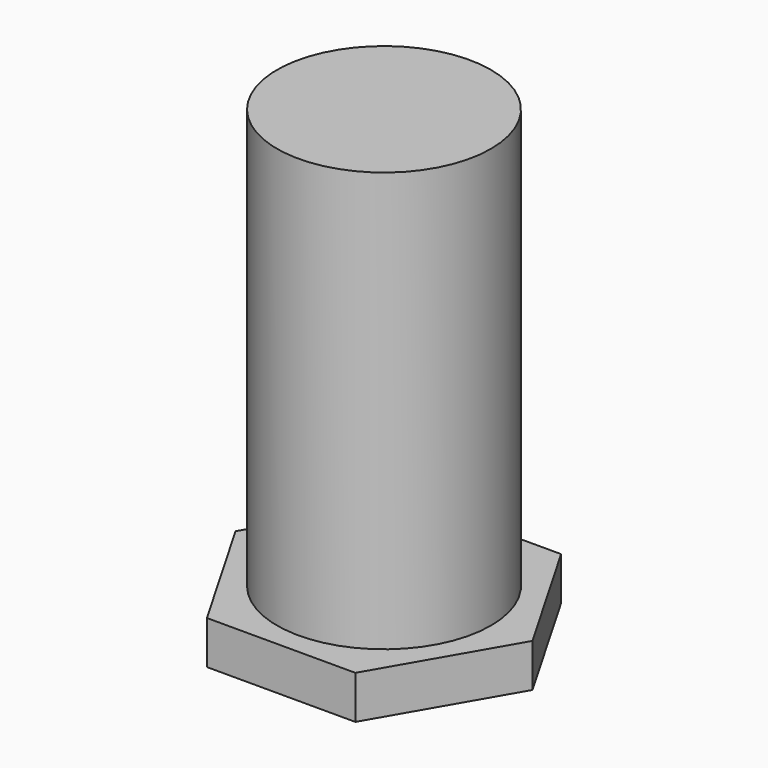
from build123d import *

# Parameters (mm, degrees)
F1_DEPTH = 1.6002
F2_R     = 3.9624
F3_DEPTH = 15.5448
F5_D     = 4.7244
F5_DEPTH = 10.922
F5_TIP   = 1.4193529543


# Not quite as in the source:
# - a feature names something its author has since deleted; it is built from what else it names


with BuildPart() as f1:
    # F0 (on Top) → F1 (new body)
    with BuildSketch(Plane.XY):
        Polygon((5.4991, 0), (2.74955, 4.762360298), (-2.74955, 4.762360298), (-5.4991, 0), (-2.74955, -4.762360298), (2.74955, -4.762360298), align=None)
    extrude(amount=F1_DEPTH)

    # F2 (on face) → F3 (join)
    with BuildSketch(Plane.XY.offset(1.6002)):
        Circle(F2_R)
    extrude(amount=F3_DEPTH)

    # F5
    with Locations(Plane(origin=(0, 0, 0), x_dir=(1, 0, 0), z_dir=(0, 0, -1))):
        with Locations((0, 0)):
            Hole(F5_D / 2, depth=F5_DEPTH)
            with Locations((0, 0, -(F5_DEPTH + F5_TIP / 2))):  # 118° drill point
                Cone(0, F5_D / 2, F5_TIP, mode=Mode.SUBTRACT)


solid = f1.part
